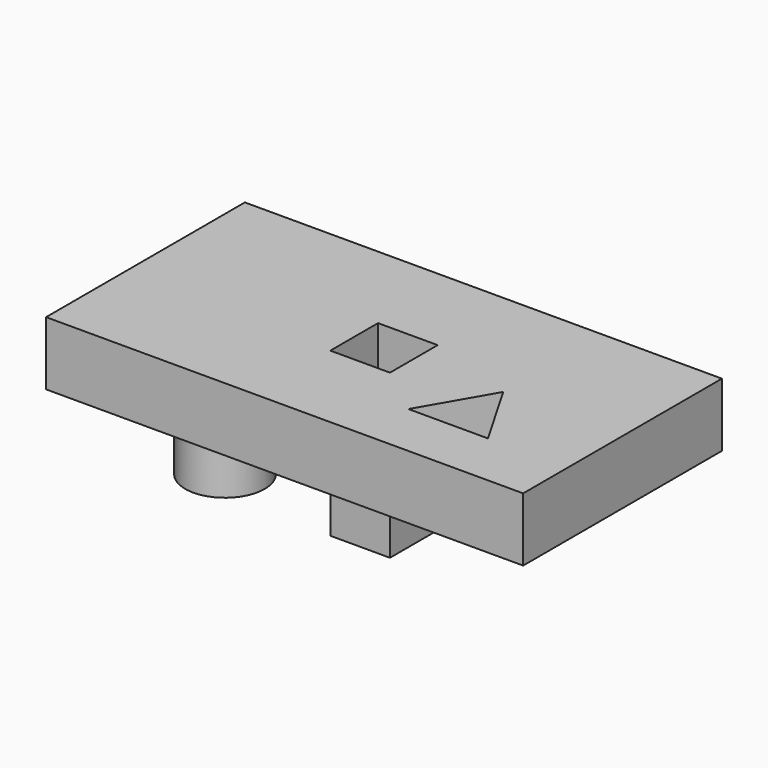
from build123d import *

# Parameters (mm, degrees)
F0_W     = 152.4
F0_H     = 79.375
F0_R     = 12.7
F0_W_2   = 19.05
F0_H_2   = 19.05
F1_DEPTH = 20.32
F2_DEPTH = 31.75
F3_DEPTH = 31.75


# Not quite as in the source:
# - a feature names something its author has since deleted; it is built from what else it names


with BuildPart() as f1:
    # F0 (on Top) → F1 (new body)
    with BuildSketch(Plane.XY):
        with Locations((-31.75, 0)):
            Rectangle(F0_W, F0_H)
        Polygon((-6.35, -21.9970452561), (6.35, 0), (19.05, -21.9970452561), align=None, mode=Mode.SUBTRACT)
        with Locations((-82.55, 0)):
            Circle(F0_R, mode=Mode.SUBTRACT)
        with Locations((-31.75, 0)):
            Rectangle(F0_W_2, F0_H_2, mode=Mode.SUBTRACT)
        with Locations((-82.55, 0)):
            Circle(F0_R)
    extrude(amount=F1_DEPTH)


with BuildPart() as f2:
    # F0 (on Top) → F2 (new body)
    with BuildSketch(Plane.XY):
        with Locations((-82.55, 0)):
            Circle(F0_R)
    extrude(amount=-F2_DEPTH)


with BuildPart() as f3:
    # F0 (on Top) → F3 (new body)
    with BuildSketch(Plane.XY):
        with Locations((-31.75, 0)):
            Rectangle(F0_W_2, F0_H_2)
    extrude(amount=-F3_DEPTH)


solid = Compound([f1.part, f2.part, f3.part])
